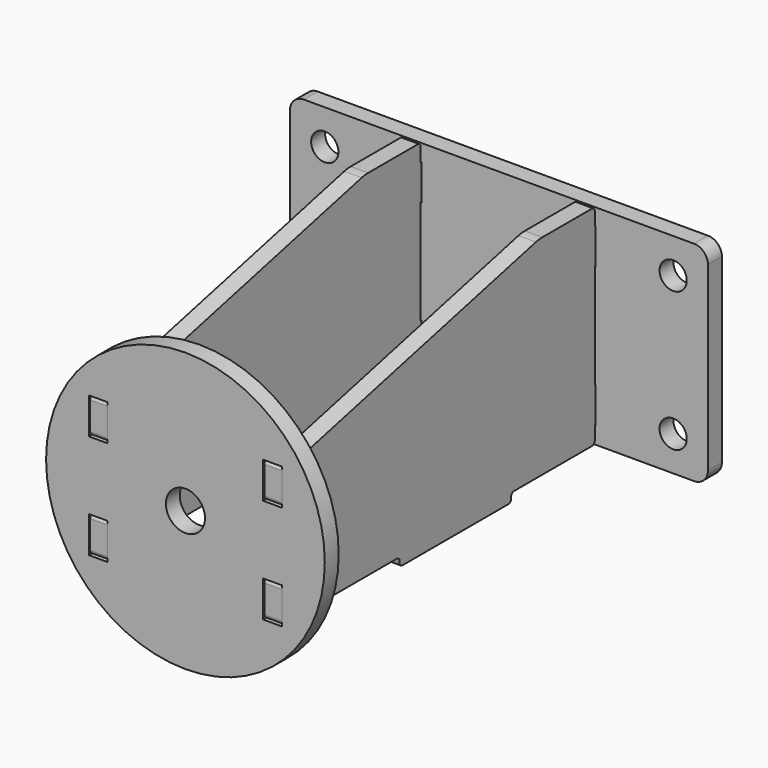
from build123d import *

# Parameters (mm, degrees)
F0_R      = 50.8
F0_R_2    = 7.1374
F0_W      = 6.35
F0_H      = 24.892
F1_DEPTH  = 6.35
F0_H_2    = 12.7
F0_H_3    = 0.254
F2_DEPTH  = 136.525
F3_DEPTH  = 6.096
F5_DEPTH  = 6.35
F6_W      = 6.35
F6_H      = 12.7
F7_DEPTH  = 6.096
F8_R      = 1.27
F9_R      = 12.7
F10_W     = 76.2
F10_H     = 76.2
F10_W_2   = 6.858
F10_H_2   = 13.208
F10_R     = 4.9657
F11_DEPTH = 6.35
F12_R     = 5.08
F15_W     = 50.8
F15_H     = 3.175
F16_DEPTH = 6.35
F17_DEPTH = 6.35
F18_R     = 1.27


# Not quite as in the source:
# - a feature names something its author has since deleted; it is built from what else it names


with BuildPart() as f1:
    # F0 (on Front) → F1 (new body)
    with BuildSketch(Plane.XZ):
        Circle(F0_R)
        Polygon((-28.321, 12.446), (-28.575, 12.446), (-28.575, -12.446), (-28.321, -12.446), (-28.321, -25.654), (-35.179, -25.654), (-35.179, -12.446), (-34.925, -12.446), (-34.925, 12.446), (-35.179, 12.446), (-35.179, 25.654), (-28.321, 25.654), align=None, mode=Mode.SUBTRACT)
        Circle(F0_R_2, mode=Mode.SUBTRACT)
        Polygon((28.575, -12.446), (28.575, 12.446), (28.321, 12.446), (28.321, 25.654), (35.179, 25.654), (35.179, 12.446), (34.925, 12.446), (34.925, -12.446), (35.179, -12.446), (35.179, -25.654), (28.321, -25.654), (28.321, -12.446), align=None, mode=Mode.SUBTRACT)
        with Locations((-31.75, 0)):
            Rectangle(F0_W, F0_H)
        with Locations((31.75, 0)):
            Rectangle(F0_W, F0_H)
    extrude(amount=F1_DEPTH)


with BuildPart() as f2:
    # F0 (on Front) → F2 (new body)
    with BuildSketch(Plane.XZ):
        with Locations((31.75, 19.05)):
            Rectangle(F0_W, F0_H_2)
        with Locations((31.75, 0)):
            Rectangle(F0_W, F0_H)
        with Locations((31.75, -19.05)):
            Rectangle(F0_W, F0_H_2)
        with Locations((31.75, 12.573)):
            Rectangle(F0_W, F0_H_3)
        with Locations((31.75, -12.573)):
            Rectangle(F0_W, F0_H_3)
    extrude(amount=-F2_DEPTH)

    # F0 (on Front) → F3 (join)
    with BuildSketch(Plane.XZ):
        with Locations((31.75, 19.05)):
            Rectangle(F0_W, F0_H_2)
        with Locations((31.75, -19.05)):
            Rectangle(F0_W, F0_H_2)
    extrude(amount=F3_DEPTH)

    # F4 (on face) → F5 (join)
    with BuildSketch(Plane.YZ.offset(34.925)):
        Polygon((3.9036273956, 25.4), (136.525, 25.4), (136.525, 50.8), (111.125, 50.8), align=None)
    extrude(amount=-F5_DEPTH)

    # F6 (on face) → F7 (join)
    with BuildSketch(Plane(origin=(0, 136.525, 0), x_dir=(-1, 0, 0), z_dir=(0, 1, 0))):
        with Locations((-31.75, 38.1)):
            Rectangle(F6_W, F6_H)
        with Locations((-31.75, -12.7)):
            Rectangle(F6_W, F6_H)
    extrude(amount=F7_DEPTH)

    # F8
    f8_edges = [f2.edges().sort_by_distance(p)[0] for p in [
        (31.75, -6.096, 25.4),
        (31.75, -6.096, 12.7),
        (31.75, -6.096, -12.7),
        (31.75, -6.096, -25.4),
        (31.75, 142.621, -19.05),
        (31.75, 142.621, -6.35),
        (31.75, 142.621, 31.75),
        (31.75, 142.621, 44.45),
        (31.75, 136.525, -25.4),
        (31.75, 136.525, 50.8),
    ]]
    fillet(f8_edges, radius=F8_R)

    # F9
    f9_edges = [f2.edges().sort_by_distance(p)[0] for p in [
        (31.75, 3.903627, 25.4),
        (31.75, 111.125, 50.8),
    ]]
    fillet(f9_edges, radius=F9_R)


with BuildPart() as f11:
    # F10 (on face) → F11 (new body)
    with BuildSketch(Plane(origin=(0, 142.621, 0), x_dir=(-1, 0, 0), z_dir=(0, 1, 0))):
        with Locations((38.1, 12.7)):
            Rectangle(F10_W, F10_H)
        with Locations((31.75, -12.7)):
            Rectangle(F10_W_2, F10_H_2, mode=Mode.SUBTRACT)
        with Locations((63.5, -12.7)):
            Circle(F10_R, mode=Mode.SUBTRACT)
        with Locations((31.75, 38.1)):
            Rectangle(F10_W_2, F10_H_2, mode=Mode.SUBTRACT)
        with Locations((63.5, 38.1)):
            Circle(F10_R, mode=Mode.SUBTRACT)
        with Locations((-38.1, 12.7)):
            Rectangle(F10_W, F10_H)
        with Locations((-63.5, -12.7)):
            Circle(F10_R, mode=Mode.SUBTRACT)
        with Locations((-31.75, -12.7)):
            Rectangle(F10_W_2, F10_H_2, mode=Mode.SUBTRACT)
        with Locations((-63.5, 38.1)):
            Circle(F10_R, mode=Mode.SUBTRACT)
        with Locations((-31.75, 38.1)):
            Rectangle(F10_W_2, F10_H_2, mode=Mode.SUBTRACT)
    extrude(amount=-F11_DEPTH)

    # F12
    f12_edges = [f11.edges().sort_by_distance(p)[0] for p in [
        (76.2, 139.446, 50.8),
        (76.2, 139.446, -25.4),
        (-76.2, 139.446, -25.4),
        (-76.2, 139.446, 50.8),
    ]]
    fillet(f12_edges, radius=F12_R)


with BuildPart() as f13_1:
    # F13: instance of F2
    add(f2.part.mirror(Plane.YZ))


with BuildPart() as f11_1:
    # F14: moved
    add(f11.part.moved(Location((0, 0.254, 0))))


with BuildPart() as f2_1:
    add(f2.part)

    # F15 (on face) → F16 (join)
    with BuildSketch(Plane.YZ.offset(34.925)):
        with Locations((73.025, -26.9875)):
            Rectangle(F15_W, F15_H)
    extrude(amount=-F16_DEPTH)

    # F15 (on face) → F17 (join)
    with BuildSketch(Plane.YZ.offset(34.925)):
        with Locations((73.025, -26.9875)):
            Rectangle(F15_W, F15_H)
    extrude(amount=-F17_DEPTH)

    # F18
    f18_edges = [f2_1.edges().sort_by_distance(p)[0] for p in [
        (31.75, 47.625, -28.575),
        (31.75, 98.425, -28.575),
        (31.75, 98.425, -25.4),
        (31.75, 47.625, -25.4),
    ]]
    fillet(f18_edges, radius=F18_R)


with BuildPart() as f19_1:
    # F19: instance of F2
    add(f2_1.part.mirror(Plane.YZ))


with BuildPart() as f22_1:
    # F22: instance of F2
    add(f2_1.part.mirror(Plane.YZ))


solid = Compound([f1.part, f11_1.part, f2_1.part, f22_1.part])
